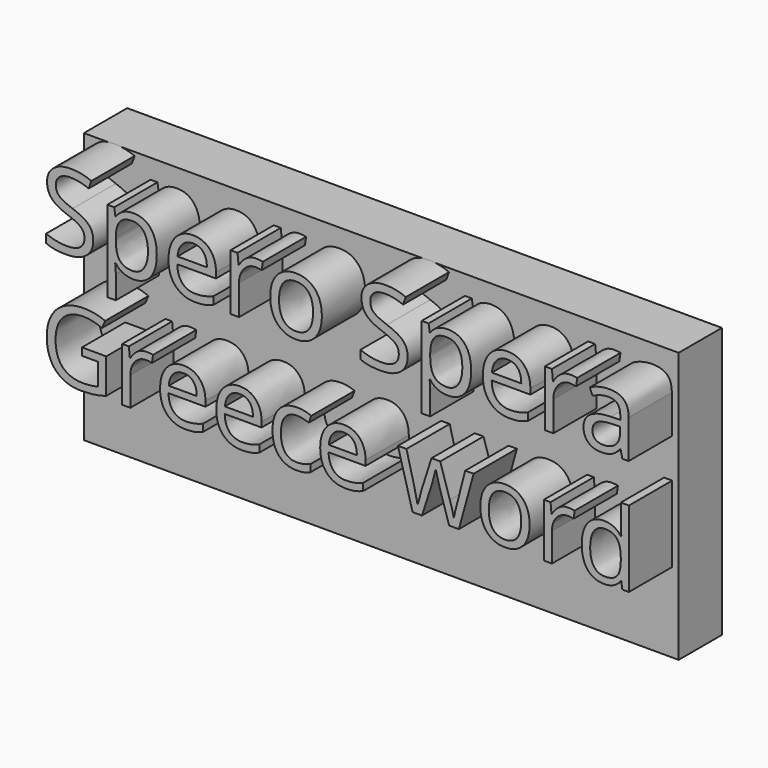
from build123d import *

# Parameters (mm, degrees)
F0_W         = 55
F0_H         = 25
F1_DEPTH     = 5
F2_TEXT_SIZE = 9.7068637454
F3_DEPTH     = 5
F4_TEXT_SIZE = 9.2634016685
F5_DEPTH     = 5


# Not quite as in the source:
# - Text() gives the source's letters only with a copy of the font that has no kerning and outlines rounded to 1/6400 em; it was checked with that copy


with BuildPart() as f1:
    # F0 (on Front) → F1 (new body)
    with BuildSketch(Plane.XZ):
        with Locations((27.5, 12.5)):
            Rectangle(F0_W, F0_H)
    extrude(amount=F1_DEPTH)

    # F2 (on face) → F3 (join)
    with BuildSketch(Plane.XZ.offset(5)):
        with Locations((0, 18.0110581033)):
            Text('Spero Spera', F2_TEXT_SIZE, font='Open Sans', text_align=(TextAlign.LEFT, TextAlign.BOTTOM))
    extrude(amount=F3_DEPTH)

    # F4 (on face) → F5 (join)
    with BuildSketch(Plane.XZ.offset(5)):
        with Locations((0, 7.3634773186)):
            Text('Greece word', F4_TEXT_SIZE, font='Open Sans', text_align=(TextAlign.LEFT, TextAlign.BOTTOM))
    extrude(amount=F5_DEPTH)


solid = f1.part
